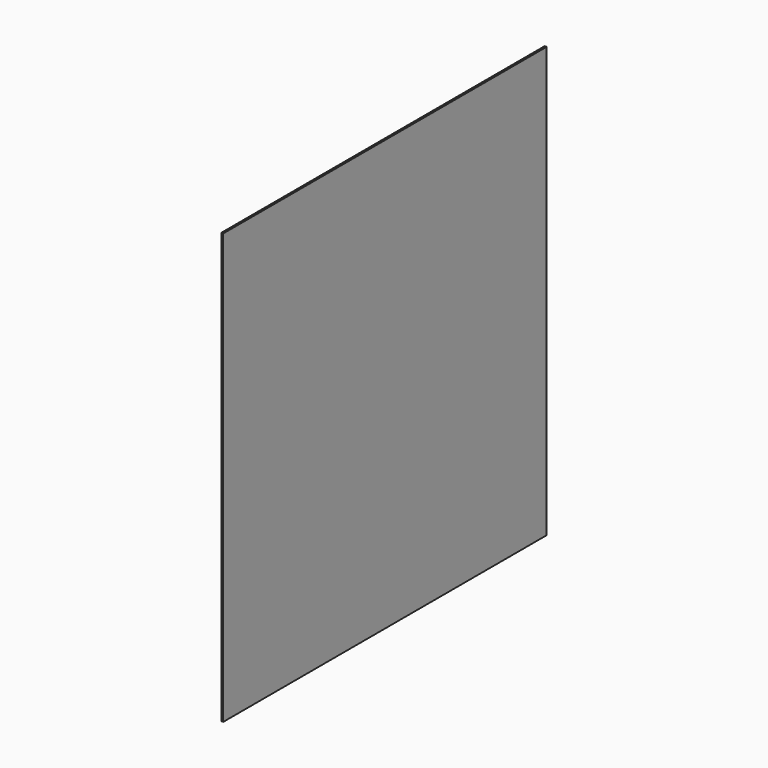
from build123d import *

# Parameters (mm, degrees)
F0_W     = 630
F0_H     = 670
F1_DEPTH = 3


# Not quite as in the source:
# - the program builds the solid bodies; features that only make, move or delete a surface that nothing else refers to are left out


with BuildPart() as f1:
    # F0 (on Right) → F1 (new body)
    with BuildSketch(Plane.YZ):
        Rectangle(F0_W, F0_H)
    extrude(amount=F1_DEPTH)


solid = f1.part
